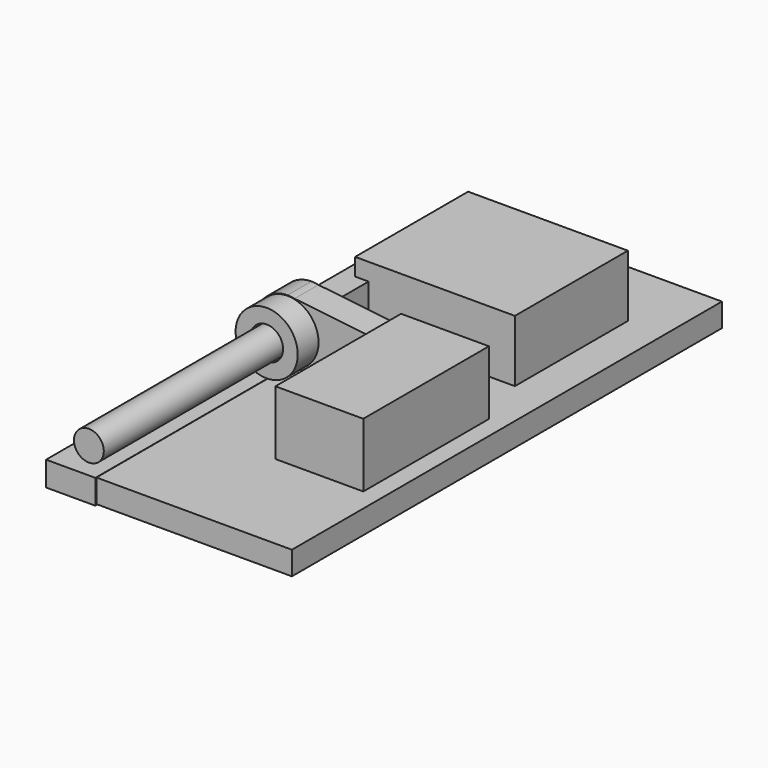
from build123d import *

# Parameters (mm, degrees)
F0_R      = 14.3293647742
F0_R_2    = 8.090753617
F1_DEPTH  = 25.4459455609
F2_R      = 26.470860224
F2_R_2    = 13.9856812783
F3_DEPTH  = 47.6294439286
F4_R      = 13.4706024235
F4_R_2    = 7.084059424
F5_DEPTH  = 38.3975785226
F6_R      = 12.7
F7_DEPTH  = 236.9658201933
F8_R      = 7.6266251534
F9_DEPTH  = 38.9788094908
F10_W     = 457.9400420189
F10_H     = 19.9817121029
F11_DEPTH = 166.583776474
F14_W     = 120.3324198723
F14_H     = 52.7262985706
F15_DEPTH = 136.1045930535
F16_W     = 460.1263403893
F16_H     = 20.917981863
F17_DEPTH = 41.9985167682
F18_W     = 22.9237377644
F18_H     = 23.126155138
F19_DEPTH = 65.294874832
F22_R     = 5.7126926056
F23_DEPTH = 72.8688146919
F24_W     = 74.8696923256
F24_H     = 54.8530220985
F25_DEPTH = 133.7927896529


# Not quite as in the source:
# - the program builds the solid bodies; features that only make, move or delete a surface that nothing else refers to are left out


with BuildPart() as f1:
    # F0 (on Front) → F1 (new body)
    with BuildSketch(Plane.XZ):
        with BuildLine():
            Line((5.9606575044, 26.2333161817), (0, 26.901976057))
            ThreePointArc((0, 26.901976057), (-26.901976057, 0), (0, -26.901976057))
            Line((0, -26.901976057), (5.9606575044, -26.2333161817))
            ThreePointArc((5.9606575044, -26.2333161817), (21.024625814, -16.7833675153), (26.901976057, 0))
            ThreePointArc((26.901976057, 0), (21.024625814, 16.7833675153), (5.9606575044, 26.2333161817))
        make_face()
        Circle(F0_R, mode=Mode.SUBTRACT)
        with BuildLine():
            ThreePointArc((5.9606575044, 26.2333161817), (2.9990225038, 26.7342884662), (0, 26.901976057))
            Line((0, 26.901976057), (5.9606575044, 26.2333161817))
        make_face()
        with BuildLine():
            Line((5.9606575044, -26.2333161817), (0, -26.901976057))
            ThreePointArc((0, -26.901976057), (2.9990225038, -26.7342884662), (5.9606575044, -26.2333161817))
        make_face()
        with BuildLine():
            Line((114.7026486896, 14.0347615394), (5.9606575044, 26.2333161817))
            ThreePointArc((5.9606575044, 26.2333161817), (21.024625814, 16.7833675153), (26.901976057, 0))
            ThreePointArc((26.901976057, 0), (21.024625814, -16.7833675153), (5.9606575044, -26.2333161817))
            Line((5.9606575044, -26.2333161817), (114.7026486896, -14.0347615394))
            ThreePointArc((114.7026486896, -14.0347615394), (99.0054519932, 0), (114.7026486896, 14.0347615394))
        make_face()
        with BuildLine():
            ThreePointArc((127.2510377605, 0), (123.6564987159, 9.4132433271), (114.7026486896, 14.0347615394))
            ThreePointArc((114.7026486896, 14.0347615394), (99.0054519932, 0), (114.7026486896, -14.0347615394))
            ThreePointArc((114.7026486896, -14.0347615394), (123.6564987159, -9.4132433271), (127.2510377605, 0))
        make_face()
        with Locations((113.1282448769, 0)):
            Circle(F0_R_2, mode=Mode.SUBTRACT)
    extrude(amount=F1_DEPTH)

    # F2 (on Front) → F3 (join)
    with BuildSketch(Plane.XZ):
        Circle(F2_R)
        Circle(F2_R_2, mode=Mode.SUBTRACT)
    extrude(amount=F3_DEPTH)

    # F4 (on Front) → F5 (join)
    with BuildSketch(Plane.XZ):
        with Locations((113.1200492382, 0)):
            Circle(F4_R)
        with Locations((113.1200492382, 0)):
            Circle(F4_R_2, mode=Mode.SUBTRACT)
    extrude(amount=F5_DEPTH)


with BuildPart() as f7:
    # F6 (on Front) → F7 (new body)
    with BuildSketch(Plane.XZ):
        Circle(F6_R)
    extrude(amount=F7_DEPTH)

    # F8 (on Front) → F9 (join)
    with BuildSketch(Plane.XZ):
        Circle(F8_R)
    extrude(amount=-F9_DEPTH)


with BuildPart() as f11:
    # F10 (on Right) → F11 (new body)
    with BuildSketch(Plane.YZ):
        with Locations((0, -37.1216386557)):
            Rectangle(F10_W, F10_H)
    extrude(amount=F11_DEPTH)

    # F16 (on Right) → F17 (join)
    with BuildSketch(Plane.YZ):
        with Locations((0, -37.4110639095)):
            Rectangle(F16_W, F16_H)
    extrude(amount=-F17_DEPTH)


with BuildPart() as f15:
    # F14 (on Right) → F15 (new body)
    with BuildSketch(Plane.YZ):
        with Locations((106.7316830158, 0)):
            Rectangle(F14_W, F14_H)
    extrude(amount=F15_DEPTH)


with BuildPart() as f19:
    # F18 (on Front) → F19 (new body)
    with BuildSketch(Plane.XZ):
        Rectangle(F18_W, F18_H)
    extrude(amount=-F19_DEPTH)


with BuildPart() as f23:
    # F22 (on Front) → F23 (new body)
    with BuildSketch(Plane.XZ):
        with Locations((113.857075572, 0)):
            Circle(F22_R)
    extrude(amount=F23_DEPTH)


with BuildPart() as f25:
    # F24 (on Front) → F25 (new body)
    with BuildSketch(Plane.XZ):
        with Locations((113.8191521168, 0)):
            Rectangle(F24_W, F24_H)
    extrude(amount=F25_DEPTH)


solid = Compound([f1.part, f7.part, f11.part, f15.part, f19.part, f23.part, f25.part])
